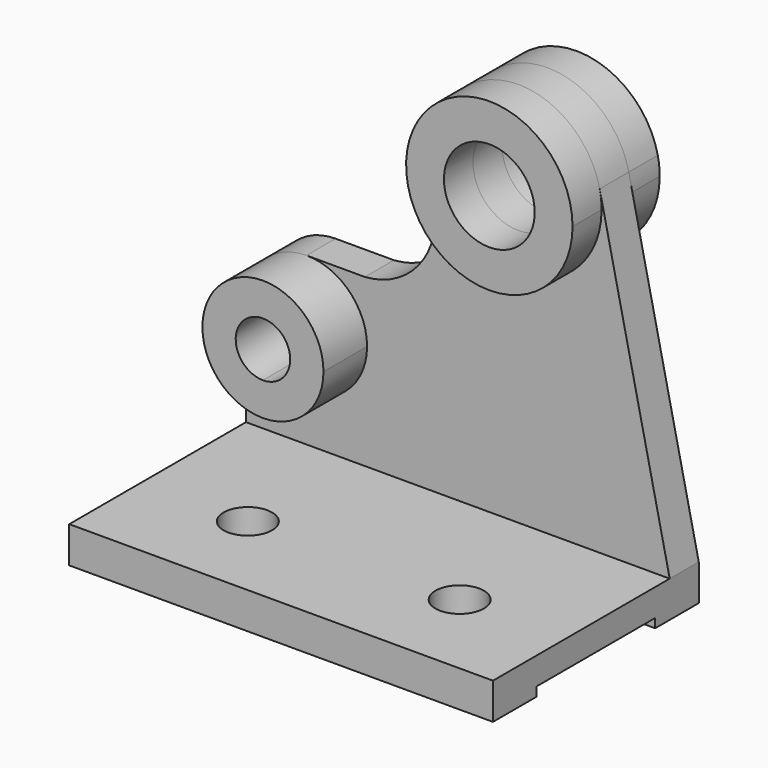
from build123d import *
from build123d import SkipClean  # not in build123d's __all__

# Parameters (mm, degrees)
F0_W      = 140
F0_H      = 85
F0_R      = 8
F1_DEPTH  = 12
F2_W      = 140
F2_H      = 12
F3_DEPTH  = 130
F5_DEPTH  = 18
F7_DEPTH  = 12
F9_DEPTH  = 25
F10_DEPTH = 25
F11_W     = 49
F11_H     = 3
F12_DEPTH = 140.001


# Not quite as in the source:
# - after a boolean that leaves OpenCascade's solid faulty, fix() repairs it
# - a feature of the source that left no trace in its solid (it failed there, or was rolled back) is left out
# - a pattern or mirror of a feature is missing from the dataset's text; its kind, count and spacing are read off the source's solid


with BuildPart() as f1:
    # F0 (on Top) → F1 (new body)
    with BuildSketch(Plane.XY):
        with Locations((70, 42.5)):
            Rectangle(F0_W, F0_H)
        with Locations((35, 30)):
            Circle(F0_R, mode=Mode.SUBTRACT)
        with Locations((105, 30)):
            Circle(F0_R, mode=Mode.SUBTRACT)
    extrude(amount=F1_DEPTH)

    # F2 (on face) → F3 (join)
    with BuildSketch(Plane.XY.offset(12)):
        with Locations((70, 79)):
            Rectangle(F2_W, F2_H)
    extrude(amount=F3_DEPTH)

    # F4 (on face) → F5 (join)
    with BuildSketch(Plane.XZ.offset(-73)):
        with BuildLine():
            ThreePointArc((40, 47), (20, 67), (0, 47))
            ThreePointArc((0, 47), (5.8578643763, 32.8578643763), (20, 27))
            ThreePointArc((20, 27), (34.1421356237, 32.8578643763), (40, 47))
        make_face()
        with BuildLine():
            ThreePointArc((29, 47), (26.3639610307, 40.6360389693), (20, 38))
            ThreePointArc((20, 38), (13.6360389693, 53.3639610307), (29, 47))
        make_face(mode=Mode.SUBTRACT)
    extrude(amount=F5_DEPTH)

    # F6 (on face) → F7 (join)
    with BuildSketch(Plane.XZ.offset(-73)):
        with BuildLine():
            ThreePointArc((117.5, 112), (70.5545635174, 131.4454364826), (90, 84.5))
            ThreePointArc((90, 84.5), (109.4454364826, 92.5545635174), (117.5, 112))
        make_face()
        with BuildLine():
            ThreePointArc((105, 112), (100.6066017178, 101.3933982822), (90, 97))
            ThreePointArc((90, 97), (79.3933982822, 122.6066017178), (105, 112))
        make_face(mode=Mode.SUBTRACT)
    f7 = extrude(amount=F7_DEPTH)

    # F7_copies: F7 across plane
    add(f7.mirror(Plane.ZX.offset(79)), clean=False)

    # F8 (on face) → F9 (cut)
    with BuildSketch(Plane.XZ.offset(-73)):
        with BuildLine():
            Line((62.5, 89.5), (62.5, 112))
            ThreePointArc((62.5, 112), (87.0476647591, 139.3410628291), (116.8660884819, 117.8705442409))
            Line((116.8660884819, 117.8705442409), (140, 12))
            Line((140, 12), (140, 142))
            Line((140, 142), (0, 142))
            Line((0, 142), (0, 47))
            ThreePointArc((0, 47), (5.8578643763, 61.1421356237), (20, 67))
            Line((20, 67), (35.9839461744, 67))
            Line((35.9839461744, 67), (39.2560265726, 67))
            ThreePointArc((39.2560265726, 67), (55.0078493135, 73.9836089388), (62.5, 89.5))
        make_face()
    with SkipClean():  # cleaning this boolean's faces spoils the solid; the shape is the same uncleaned
        extrude(amount=-F9_DEPTH, mode=Mode.SUBTRACT)

    # F10 (cut): faces of the model
    f10_faces = [f1.faces().sort_by_distance(p)[0] for p in [
        (90, 73, 112),
        (20, 73, 47),
    ]]
    extrude(f10_faces, amount=-F10_DEPTH, mode=Mode.SUBTRACT)

    add(f1.part.fix(), mode=Mode.REPLACE)

    # F11 (on face) → F12 (cut, through all)
    with BuildSketch(Plane(origin=(0, 0, 0), x_dir=(0, -1, 0), z_dir=(-1, 0, 0))):
        with Locations((-42.5, 1.5)):
            Rectangle(F11_W, F11_H)
    extrude(amount=-F12_DEPTH, mode=Mode.SUBTRACT)


solid = f1.part
